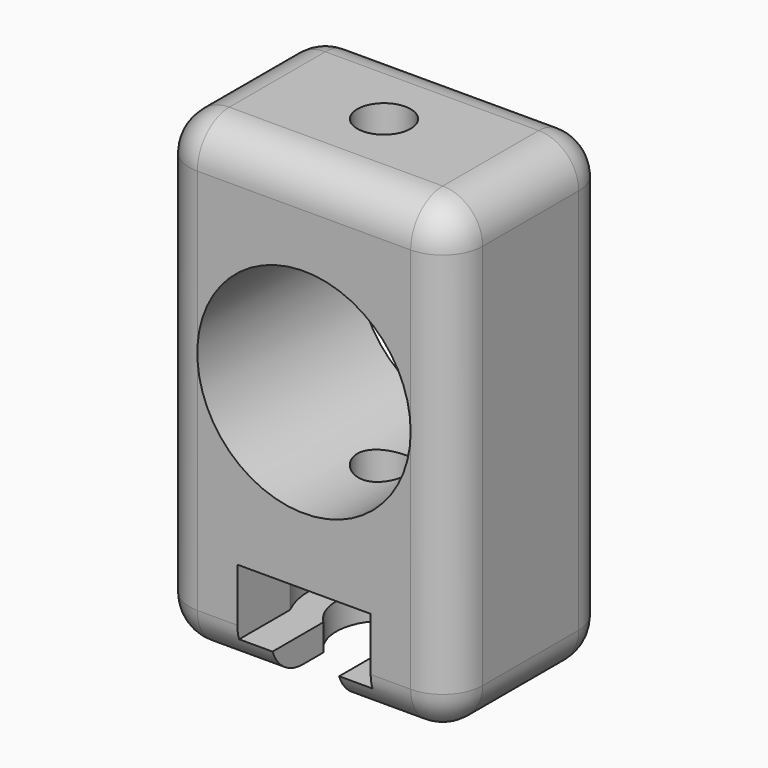
from build123d import *

# Parameters (mm, degrees)
F0_W     = 22
F0_H     = 35
F0_R     = 8
F1_DEPTH = 7.5
F3_DEPTH = 2
F6_DEPTH = 5
F7_R     = 2
F8_DEPTH = 35.001
F9_R     = 2.99999


# Not quite as in the source:
# - a fillet or chamfer is up to 0.001 mm smaller than in the source, because OpenCascade refuses the exact size


with BuildPart() as f1:
    # F0 (on Front) → F1 (new body, symmetric)
    with BuildSketch(Plane.XZ):
        with Locations((0, -2.5)):
            Rectangle(F0_W, F0_H)
        Circle(F0_R, mode=Mode.SUBTRACT)
    extrude(amount=F1_DEPTH, both=True)

    # F2 (on face) → F3 (cut)
    with BuildSketch(Plane(origin=(0, 0, -20), x_dir=(1, 0, 0), z_dir=(0, 0, -1))):
        with BuildLine():
            Line((2.5, 7.5), (-2.5, 7.5))
            Line((-2.5, 7.5), (-2.5, 2.5583377574))
            ThreePointArc((-2.5, 2.5583377574), (0, -3.5770227957), (2.5, 2.5583377574))
            Line((2.5, 2.5583377574), (2.5, 7.5))
        make_face()
    extrude(amount=-F3_DEPTH, mode=Mode.SUBTRACT)

    # F5 (on offset) → F6 (cut)
    with BuildSketch(Plane(origin=(0, 0, -18), x_dir=(1, 0, 0), z_dir=(0, 0, -1))):
        with BuildLine():
            Line((5, 7.5), (-5, 7.5))
            Line((-5, 7.5), (-5, 2.5583377574))
            ThreePointArc((-5, 2.5583377574), (0, -5.6165017654), (5, 2.5583377574))
            Line((5, 2.5583377574), (5, 7.5))
        make_face()
    extrude(amount=-F6_DEPTH, mode=Mode.SUBTRACT)

    # F7 (on face) → F8 (cut, through all)
    with BuildSketch(Plane.XY.offset(15)):
        Circle(F7_R)
    extrude(amount=-F8_DEPTH, mode=Mode.SUBTRACT)

    # F9 (radius 3 in the source; OpenCascade refuses exactly that, so slightly less here)
    f9_edges = [f1.edges().sort_by_distance(p)[0] for p in [
        (-11, 0, 15),
        (11, 0, 15),
        (0, -7.5, 15),
        (0, 7.5, 15),
        (11, -7.5, -2.5),
        (-11, -7.5, -2.5),
        (-11, 7.5, -2.5),
        (11, 7.5, -2.5),
        (0, 7.5, -20),
        (-6.75, -7.5, -20),
        (6.75, -7.5, -20),
        (-11, 0, -20),
        (11, 0, -20),
    ]]
    fillet(f9_edges, radius=F9_R)


solid = f1.part
